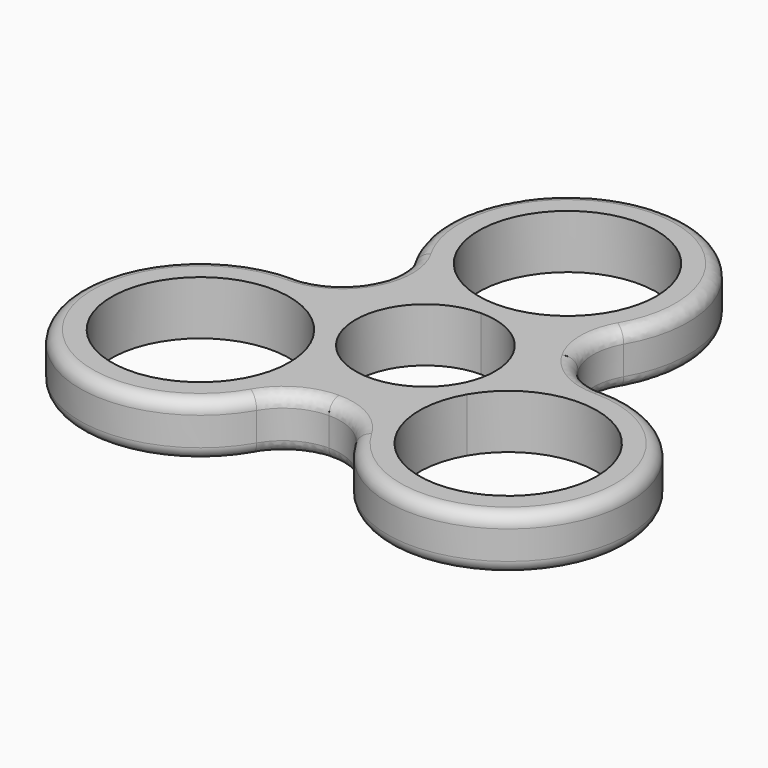
from build123d import *

# Parameters (mm, degrees)
F1_DEPTH = 8.5
F2_R     = 8.999
F3_R     = 2


# Not quite as in the source:
# - a fillet or chamfer is up to 0.001 mm smaller than in the source, because OpenCascade refuses the exact size


with BuildPart() as f1:
    # F0 (on Top) → F1 (new body)
    with BuildSketch(Plane.XY):
        with BuildLine():
            ThreePointArc((18.5469719423, 4.1242977306), (16.4544826719, 9.5), (12.8452325787, 14))
            ThreePointArc((12.8452325787, 14), (0, 47), (-12.8452325787, 14))
            ThreePointArc((-12.8452325787, 14), (-16.4544826719, 9.5), (-18.5469719423, 4.1242977306))
            ThreePointArc((-18.5469719423, 4.1242977306), (-40.7031939779, -23.5), (-5.7017393636, -18.1242977306))
            ThreePointArc((-5.7017393636, -18.1242977306), (0, -19), (5.7017393636, -18.1242977306))
            ThreePointArc((5.7017393636, -18.1242977306), (40.7031939779, -23.5), (18.5469719423, 4.1242977306))
        make_face()
        with BuildLine():
            ThreePointArc((-10.248711306, -14), (-37.771672874, -17.6234666314), (-12.124355653, -7))
            ThreePointArc((-12.124355653, -7), (-10.7257497379, -10.3765333686), (-10.248711306, -14))
        make_face(mode=Mode.SUBTRACT)
        with BuildLine():
            ThreePointArc((0, 11), (7.7781745931, 7.7781745931), (11, 0))
            ThreePointArc((11, 0), (10.6251840892, -2.8470094961), (9.5262794416, -5.5))
            ThreePointArc((9.5262794416, -5.5), (0, -11), (-9.5262794416, -5.5))
            ThreePointArc((-9.5262794416, -5.5), (-9.5262794416, 5.5), (0, 11))
        make_face(mode=Mode.SUBTRACT)
        with BuildLine():
            ThreePointArc((38.248711306, -14), (20.6252446745, -27.522961568), (12.124355653, -7))
            ThreePointArc((12.124355653, -7), (27.8721779374, -0.477038432), (38.248711306, -14))
        make_face(mode=Mode.SUBTRACT)
        with BuildLine():
            ThreePointArc((8.5917727317, 16.9464285714), (4.5414755311, 14.7570773619), (0, 14))
            ThreePointArc((0, 14), (-9.8994949366, 37.8994949366), (14, 28))
            ThreePointArc((14, 28), (12.5754685448, 21.8471477445), (8.5917727317, 16.9464285714))
        make_face(mode=Mode.SUBTRACT)
    extrude(amount=F1_DEPTH)

    # F2 (radius 9 in the source; OpenCascade refuses exactly that, so slightly less here)
    f2_edges = [f1.edges().sort_by_distance(p)[0] for p in [
        (-12.845233, 14, 4.25),
        (-18.546972, 4.124298, 4.25),
        (-5.701739, -18.124298, 4.25),
        (5.701739, -18.124298, 4.25),
        (12.845233, 14, 4.25),
        (18.546972, 4.124298, 4.25),
    ]]
    fillet(f2_edges, radius=F2_R)

    # F3
    f3_edges = [f1.edges().sort_by_distance(p)[0] for p in [
        (15.248557, 14, 8.5),
        (0, 47, 0),
    ]]
    fillet(f3_edges, radius=F3_R)


solid = f1.part
